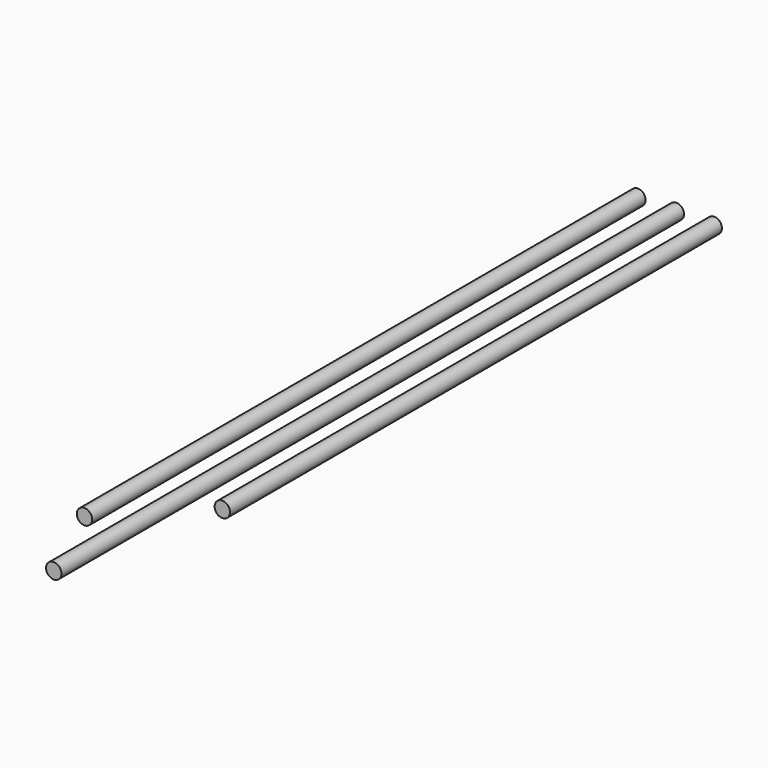
from build123d import *

# Parameters (mm, degrees)
F0_R     = 4
F1_DEPTH = 360
F2_R     = 4
F3_DEPTH = 405
F4_R     = 4
F5_DEPTH = 320


# Not quite as in the source:
# - a feature of the source that left no trace in its solid (it failed there, or was rolled back) is left out


with BuildPart() as f1:
    # F0 (on Front) → F1 (new body)
    with BuildSketch(Plane.XZ):
        Circle(F0_R)
    extrude(amount=F1_DEPTH)


with BuildPart() as f3:
    # F2 (on Front) → F3 (new body)
    with BuildSketch(Plane.XZ):
        with Locations((20.0116876513, 0)):
            Circle(F2_R)
    extrude(amount=F3_DEPTH)


with BuildPart() as f5:
    # F4 (on Front) → F5 (new body)
    with BuildSketch(Plane.XZ):
        with Locations((39.7211872041, 0)):
            Circle(F4_R)
    extrude(amount=F5_DEPTH)


solid = Compound([f1.part, f3.part, f5.part])
